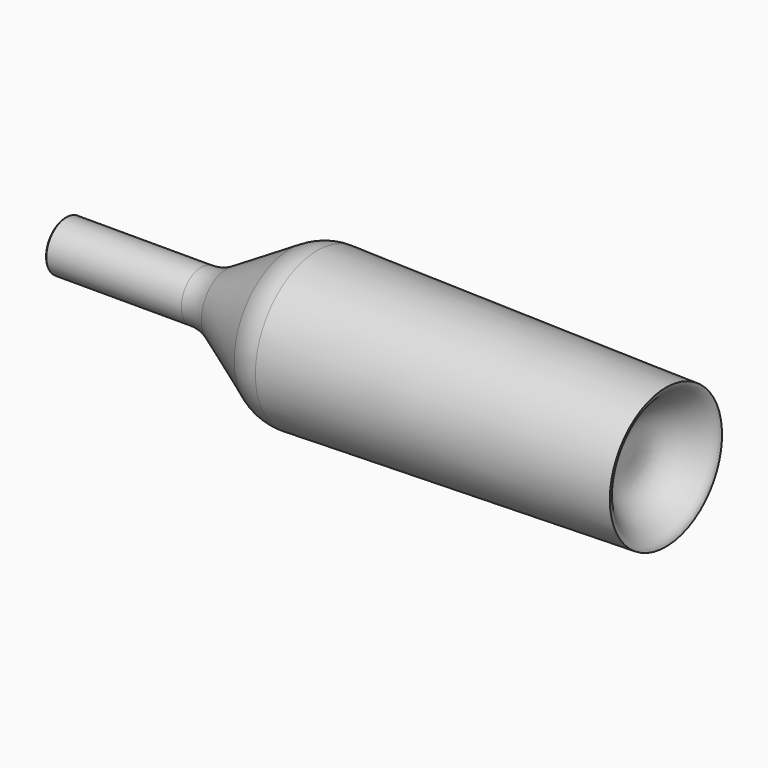
from build123d import *


# Not quite as in the source:
# - ends of sketch curves that miss each other by under 0.0002 mm in the source are joined
# - the dataset's text gives a spline's control points without its knots; the knots are read off the source's solid


with BuildPart() as f1:
    # F0 (on Top) → F1 (revolve)
    with BuildSketch(Plane.XY):
        with BuildLine():
            ThreePointArc((-285.75, -11.43), (-285.5490287786, -12.167016937), (-285.0017514707, -12.7))
            Line((-285.0017514707, -12.7), (-216.5853927097, -12.7))
            ThreePointArc((-216.5853927097, -12.7), (-209.8052797295, -13.6216408234), (-203.5172005218, -16.3196796869))
            Line((-203.5172005218, -16.3196796869), (-171.3760702521, -35.6043578488))
            ThreePointArc((-171.3760702521, -35.6043578488), (-164.8344445945, -38.3712151601), (-157.7824732637, -39.2186028951))
            Line((-157.7824732637, -39.2186028951), (19.05, -35.56))
            add(Edge.make_bspline(
                [(19.05, -35.56), (18.8199370568, -30.7601188197), (-1.2317807445, -20.8787296757), (0.1635549587, -4.0029242831), (-5.1918e-06, -1.9625883677), (0, 0)],
                knots=[0, 0, 0, 0, 0.4507733435, 0.8068049822, 1, 1, 1, 1], degree=3))
            Line((0, 0), (-2.54, 0))
            add(Edge.make_bspline(
                [(14.8285794135, -33.1067947702), (14.5353050036, -32.7990607261), (13.8691865137, -32.1447406693), (12.2944674544, -30.73758966), (9.9695334737, -28.8275639769), (7.4490348824, -26.7626250066), (5.4570185152, -25.0088190546), (4.0093053584, -23.6366363216), (2.641510283, -22.1980089148), (1.5988268496, -20.9351240128), (0.8394327936, -19.8719511734), (0.1492382006, -18.7893744625), (-0.5810765462, -17.4218736538), (-1.2672380096, -15.7774032099), (-1.9564088602, -13.6109085126), (-2.4520800573, -11.0014246266), (-2.6128292518, -8.638851289), (-2.627993734, -6.9624293235), (-2.6035900901, -5.8300997647), (-2.5708007223, -5.0090073669), (-2.547044183, -4.4386671163), (-2.5331221367, -4.0633936667), (-2.5236240841, -3.723792553), (-2.5156422476, -3.3057754423), (-2.5131648633, -2.8291110855), (-2.5181696061, -2.2621652533), (-2.530667923, -1.4312861782), (-2.5400016792, -0.6509680927), (-2.54, 0)],
                knots=[0.1260546343, 0.1260546343, 0.1260546343, 0.1260546343, 0.15625, 0.1875, 0.25, 0.3125, 0.34375, 0.375, 0.40625, 0.4375, 0.453125, 0.46875, 0.5, 0.53125, 0.5625, 0.625, 0.6875, 0.71875, 0.75, 0.78125, 0.796875, 0.8125, 0.828125, 0.84375, 0.875, 0.90625, 0.9375, 0.999999785, 0.999999785, 0.999999785, 0.999999785], degree=3))
            Line((14.8285794135, -33.1067947702), (-157.8350137437, -36.6791463592))
            ThreePointArc((-157.8350137437, -36.6791463592), (-164.1817879415, -35.9164973976), (-170.0692510333, -33.4263258174))
            Line((-170.0692510333, -33.4263258174), (-202.210381303, -14.1416476556))
            ThreePointArc((-202.210381303, -14.1416476556), (-209.1272684315, -11.1738049058), (-216.5853927097, -10.16))
            Line((-216.5853927097, -10.16), (-285.0017514707, -10.16))
            ThreePointArc((-285.0017514707, -10.16), (-285.5490287786, -10.692983063), (-285.75, -11.43))
        make_face()
    revolve(axis=Axis((-142.875, 0, 0), (-1, 0, 0)))


solid = f1.part
